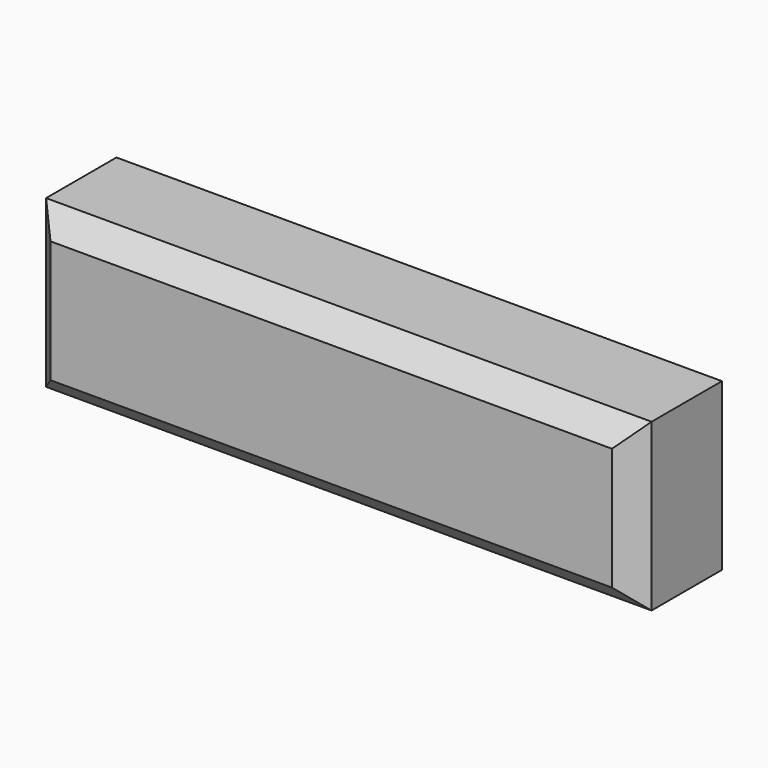
from build123d import *

# Parameters (mm, degrees)
F0_W     = 139.9047672749
F0_H     = 38.4024083614
F1_DEPTH = 12.7
F2_DEPTH = 12.7
F3_SIZE  = 5.08


# Not quite as in the source:
# - the program builds the solid bodies; features that only make, move or delete a surface that nothing else refers to are left out


with BuildPart() as f1:
    # F0 (on Front) → F1 (new body)
    with BuildSketch(Plane.XZ):
        Rectangle(F0_W, F0_H)
    extrude(amount=F1_DEPTH)

    # F2 (add): a face of the model
    f2_faces = [f1.faces().sort_by_distance(p)[0] for p in [
        (0, 0, 0),
    ]]
    extrude(f2_faces, amount=F2_DEPTH)

    # F3
    f3_edges = [f1.edges().sort_by_distance(p)[0] for p in [
        (69.952384, -12.7, 0),
        (0, -12.7, 19.201204),
        (-69.952384, -12.7, 0),
        (0, -12.7, -19.201204),
    ]]
    chamfer(f3_edges, length=F3_SIZE)


solid = f1.part
